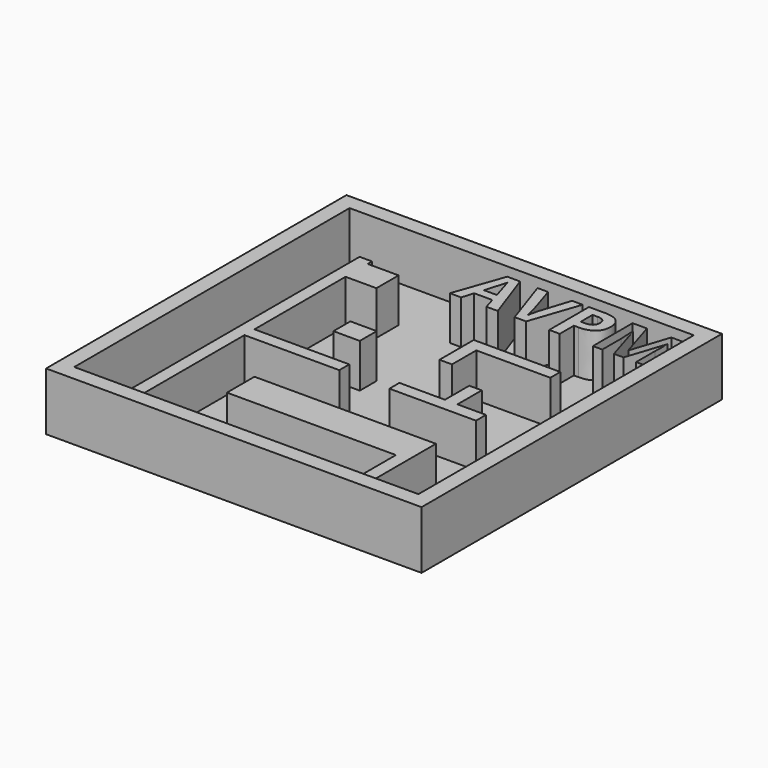
from build123d import *

# Parameters (mm, degrees)
F0_W         = 38.1
F0_H         = 38.1
F1_DEPTH     = 0.79375
F2_W         = 38.1
F2_H         = 38.1
F2_W_2       = 34.925
F2_H_2       = 34.925
F3_DEPTH     = 5.08
F4_R         = 1.27
F5_DEPTH     = 0.396875
F6_DEPTH     = 4.445
F4_TEXT_SIZE = 7.0555555556
F7_DEPTH     = 4.445
F4_W         = 2.675447613
F4_H         = 2.1494432003
F8_DEPTH     = 4.445


# Not quite as in the source:
# - a feature names something its author has since deleted; it is built from what else it names
# - Text() gives the source's letters only with a copy of the font that has no kerning and outlines rounded to 1/6400 em; it was checked with that copy


with BuildPart() as f1:
    # F0 (on Top) → F1 (new body)
    with BuildSketch(Plane.XY):
        with Locations((1.1893007904, -3.9636891358)):
            Rectangle(F0_W, F0_H)
    extrude(amount=F1_DEPTH)

    # F2 (on face) → F3 (join)
    with BuildSketch(Plane.XY.offset(0.79375)):
        with Locations((1.1893007904, -3.9636891358)):
            Rectangle(F2_W, F2_H)
        with Locations((1.1893007904, -3.9636891358)):
            Rectangle(F2_W_2, F2_H_2, mode=Mode.SUBTRACT)
    extrude(amount=F3_DEPTH)

    # F4 (on face) → F5 (cut)
    with BuildSketch(Plane.XY.offset(0.79375)):
        with Locations((-13.7331992096, -17.9566461593)):
            Circle(F4_R)
        with Locations((16.1118007904, -19.2253030837)):
            Circle(F4_R)
    extrude(amount=-F5_DEPTH, mode=Mode.SUBTRACT)

    # F4 (on face) → F6 (join)
    with BuildSketch(Plane.XY.offset(0.79375)):
        Polygon((-11.1931992096, 8.4188108642), (-11.1931992096, -21.4261891358), (-9.9231992096, -21.4261891358), (-9.9231992096, -7.7736891358), (-0.2978164961, -7.7736891358), (-0.2978164961, -6.5036891358), (-9.9231992096, -6.5036891358), (-9.9231992096, 5.0475504249), (-6.7878867096, 5.0475504249), (-6.7878867096, 7.8630140051), (-9.9231992096, 7.8630140051), (-9.9231992096, 8.4188108642), align=None)
        Polygon((4.7821835039, -6.5036891358), (4.7821835039, -7.7736891358), (13.5718007904, -7.7736891358), (13.5718007904, -6.5036891358), (10.679035556, -6.5036891358), (10.679035556, -3.4241614497), (9.409035556, -3.4241614497), (9.409035556, -6.5036891358), align=None)
        Polygon((13.5718007904, 2.9258385503), (4.7821835039, 2.9258385503), (4.7821835039, 1.6558385503), (4.7860196153, 1.6558385503), (4.7860196153, -1.4236891358), (6.0560196153, -1.4236891358), (6.0560196153, 1.6558385503), (13.5718007904, 1.6558385503), align=None)
        Polygon((12.3018007904, -16.3461891358), (12.3018007904, -21.4261891358), (13.5718007904, -21.4261891358), (13.5718007904, -16.3461891358), (13.5718007904, -12.8536891358), (12.3018007904, -12.8536891358), (-4.8431992096, -12.8536891358), (-4.8431992096, -16.3461891358), (-0.6950401003, -16.3461891358), align=None)
    extrude(amount=F6_DEPTH)

    # F4 (on face) → F7 (join)
    with BuildSketch(Plane.XY.offset(0.79375)):
        with Locations((-1.7078867096, 8.0058385503)):
            Text('AVPM', F4_TEXT_SIZE, font='Open Sans', font_style=FontStyle.BOLD, text_align=(TextAlign.LEFT, TextAlign.BOTTOM))
    extrude(amount=F7_DEPTH)

    # F4 (on face) → F8 (join)
    with BuildSketch(Plane.XY.offset(0.79375)):
        with Locations((-3.5054754031, -1.7632860399)):
            Rectangle(F4_W, F4_H)
    extrude(amount=F8_DEPTH)


solid = f1.part
